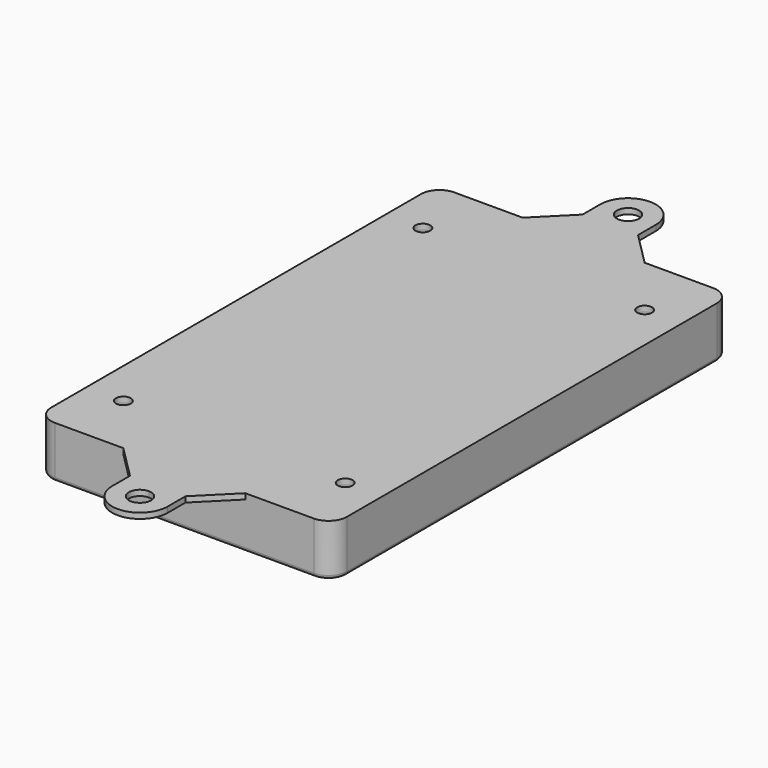
from build123d import *

# Parameters (mm, degrees)
F0_R      = 4
F1_DEPTH  = 25
F2_DEPTH  = 3
F3_DEPTH  = 18
F6_DEPTH  = 2
F8_DEPTH  = 20
F9_DEPTH  = 16
F10_DEPTH = 25
F7_R      = 6
F7_R_2    = 4
F11_DEPTH = 6
F13_DEPTH = 9
F14_R     = 3
F15_R     = 2
F16_R     = 4
F16_R_2   = 6
F17_DEPTH = 3


with BuildPart() as f1:
    # F0 (on Top) → F1 (new body)
    with BuildSketch(Plane.XY):
        with BuildLine():
            ThreePointArc((14.05, 38.3825811321), (16.9789321881, 31.3115133202), (24.05, 28.3825811321))
            Line((24.05, 28.3825811321), (164.05, 28.3825811321))
            ThreePointArc((164.05, 28.3825811321), (171.1210678119, 31.3115133202), (174.05, 38.3825811321))
            Line((174.05, 38.3825811321), (174.05, 288.3825811321))
            ThreePointArc((174.05, 288.3825811321), (171.1210678119, 295.4536489439), (164.05, 298.3825811321))
            Line((164.05, 298.3825811321), (24.05, 298.3825811321))
            ThreePointArc((24.05, 298.3825811321), (16.9789321881, 295.4536489439), (14.05, 288.3825811321))
            Line((14.05, 288.3825811321), (14.05, 38.3825811321))
        make_face()
        with Locations((34.05, 62.1325811321)):
            Circle(F0_R, mode=Mode.SUBTRACT)
        with Locations((154.05, 62.1325811321)):
            Circle(F0_R, mode=Mode.SUBTRACT)
        with Locations((34.05, 264.6325811321)):
            Circle(F0_R, mode=Mode.SUBTRACT)
        with BuildLine():
            ThreePointArc((30.05, 208.0453240566), (30.058730902, 208.5396812427), (30.0849127182, 209.033421831))
            ThreePointArc((30.0849127182, 209.033421831), (94.05, 268.6325811321), (158.0150872818, 209.033421831))
            ThreePointArc((158.0150872818, 209.033421831), (158.041269098, 208.5396812427), (158.05, 208.0453240566))
            Line((158.05, 208.0453240566), (158.05, 118.7198382075))
            ThreePointArc((158.05, 118.7198382075), (158.041269098, 118.2254810215), (158.0150872818, 117.7317404331))
            ThreePointArc((158.0150872818, 117.7317404331), (94.05, 58.1325811321), (30.0849127182, 117.7317404331))
            ThreePointArc((30.0849127182, 117.7317404331), (30.058730902, 118.2254810215), (30.05, 118.7198382075))
            Line((30.05, 118.7198382075), (30.05, 208.0453240566))
        make_face(mode=Mode.SUBTRACT)
        with Locations((154.05, 264.6325811321)):
            Circle(F0_R, mode=Mode.SUBTRACT)
        with BuildLine():
            ThreePointArc((158.0150872818, 209.033421831), (94.05, 268.6325811321), (30.0849127182, 209.033421831))
            ThreePointArc((30.0849127182, 209.033421831), (30.058730902, 208.5396812427), (30.05, 208.0453240566))
            Line((30.05, 208.0453240566), (30.05, 118.7198382075))
            ThreePointArc((30.05, 118.7198382075), (30.058730902, 118.2254810215), (30.0849127182, 117.7317404331))
            ThreePointArc((30.0849127182, 117.7317404331), (94.05, 58.1325811321), (158.0150872818, 117.7317404331))
            ThreePointArc((158.0150872818, 117.7317404331), (158.041269098, 118.2254810215), (158.05, 118.7198382075))
            Line((158.05, 118.7198382075), (158.05, 208.0453240566))
            ThreePointArc((158.05, 208.0453240566), (158.041269098, 208.5396812427), (158.0150872818, 209.033421831))
        make_face()
        with BuildLine():
            Line((34.05, 118.7198382075), (34.05, 208.0453240566))
            ThreePointArc((34.05, 208.0453240566), (34.0562363586, 208.3984363324), (34.0749376559, 208.7511081812))
            ThreePointArc((34.0749376559, 208.7511081812), (94.05, 264.6325811321), (154.0250623441, 208.7511081812))
            ThreePointArc((154.0250623441, 208.7511081812), (154.0437636414, 208.3984363324), (154.05, 208.0453240566))
            Line((154.05, 208.0453240566), (154.05, 118.7198382075))
            ThreePointArc((154.05, 118.7198382075), (154.0437636414, 118.3667259318), (154.0250623441, 118.0140540829))
            ThreePointArc((154.0250623441, 118.0140540829), (94.05, 62.1325811321), (34.0749376559, 118.0140540829))
            ThreePointArc((34.0749376559, 118.0140540829), (34.0562363586, 118.3667259318), (34.05, 118.7198382075))
        make_face(mode=Mode.SUBTRACT)
        with BuildLine():
            ThreePointArc((34.0749376559, 208.7511081812), (34.0562363586, 208.3984363324), (34.05, 208.0453240566))
            Line((34.05, 208.0453240566), (34.05, 118.7198382075))
            ThreePointArc((34.05, 118.7198382075), (34.0562363586, 118.3667259318), (34.0749376559, 118.0140540829))
            ThreePointArc((34.0749376559, 118.0140540829), (94.05, 62.1325811321), (154.0250623441, 118.0140540829))
            ThreePointArc((154.0250623441, 118.0140540829), (154.0437636414, 118.3667259318), (154.05, 118.7198382075))
            Line((154.05, 118.7198382075), (154.05, 208.0453240566))
            ThreePointArc((154.05, 208.0453240566), (154.0437636414, 208.3984363324), (154.0250623441, 208.7511081812))
            ThreePointArc((154.0250623441, 208.7511081812), (94.05, 264.6325811321), (34.0749376559, 208.7511081812))
        make_face()
        with BuildLine():
            ThreePointArc((151.0325436409, 208.5393729438), (151.045634549, 208.2925026496), (151.05, 208.0453240566))
            Line((151.05, 208.0453240566), (151.05, 118.7198382075))
            ThreePointArc((151.05, 118.7198382075), (151.045634549, 118.4726596145), (151.0325436409, 118.2257893203))
            ThreePointArc((151.0325436409, 118.2257893203), (94.05, 65.1325811321), (37.0674563591, 118.2257893203))
            ThreePointArc((37.0674563591, 118.2257893203), (37.054365451, 118.4726596145), (37.05, 118.7198382075))
            Line((37.05, 118.7198382075), (37.05, 208.0453240566))
            ThreePointArc((37.05, 208.0453240566), (37.054365451, 208.2925026496), (37.0674563591, 208.5393729438))
            ThreePointArc((37.0674563591, 208.5393729438), (94.05, 261.6325811321), (151.0325436409, 208.5393729438))
        make_face(mode=Mode.SUBTRACT)
        with BuildLine():
            Line((151.05, 118.7198382075), (151.05, 208.0453240566))
            ThreePointArc((151.05, 208.0453240566), (151.045634549, 208.2925026496), (151.0325436409, 208.5393729438))
            ThreePointArc((151.0325436409, 208.5393729438), (94.05, 261.6325811321), (37.0674563591, 208.5393729438))
            ThreePointArc((37.0674563591, 208.5393729438), (37.054365451, 208.2925026496), (37.05, 208.0453240566))
            Line((37.05, 208.0453240566), (37.05, 118.7198382075))
            ThreePointArc((37.05, 118.7198382075), (37.054365451, 118.4726596145), (37.0674563591, 118.2257893203))
            ThreePointArc((37.0674563591, 118.2257893203), (94.05, 65.1325811321), (151.0325436409, 118.2257893203))
            ThreePointArc((151.0325436409, 118.2257893203), (151.045634549, 118.4726596145), (151.05, 118.7198382075))
        make_face()
    extrude(amount=-F1_DEPTH)

    # F0 (on Top) → F2 (join)
    with BuildSketch(Plane.XY):
        with BuildLine():
            ThreePointArc((34.0749376559, 208.7511081812), (34.0562363586, 208.3984363324), (34.05, 208.0453240566))
            Line((34.05, 208.0453240566), (34.05, 118.7198382075))
            ThreePointArc((34.05, 118.7198382075), (34.0562363586, 118.3667259318), (34.0749376559, 118.0140540829))
            ThreePointArc((34.0749376559, 118.0140540829), (94.05, 62.1325811321), (154.0250623441, 118.0140540829))
            ThreePointArc((154.0250623441, 118.0140540829), (154.0437636414, 118.3667259318), (154.05, 118.7198382075))
            Line((154.05, 118.7198382075), (154.05, 208.0453240566))
            ThreePointArc((154.05, 208.0453240566), (154.0437636414, 208.3984363324), (154.0250623441, 208.7511081812))
            ThreePointArc((154.0250623441, 208.7511081812), (94.05, 264.6325811321), (34.0749376559, 208.7511081812))
        make_face()
        with BuildLine():
            ThreePointArc((151.0325436409, 208.5393729438), (151.045634549, 208.2925026496), (151.05, 208.0453240566))
            Line((151.05, 208.0453240566), (151.05, 118.7198382075))
            ThreePointArc((151.05, 118.7198382075), (151.045634549, 118.4726596145), (151.0325436409, 118.2257893203))
            ThreePointArc((151.0325436409, 118.2257893203), (94.05, 65.1325811321), (37.0674563591, 118.2257893203))
            ThreePointArc((37.0674563591, 118.2257893203), (37.054365451, 118.4726596145), (37.05, 118.7198382075))
            Line((37.05, 118.7198382075), (37.05, 208.0453240566))
            ThreePointArc((37.05, 208.0453240566), (37.054365451, 208.2925026496), (37.0674563591, 208.5393729438))
            ThreePointArc((37.0674563591, 208.5393729438), (94.05, 261.6325811321), (151.0325436409, 208.5393729438))
        make_face(mode=Mode.SUBTRACT)
    extrude(amount=F2_DEPTH)

    # F0 (on Top) → F3 (cut)
    with BuildSketch(Plane.XY):
        with BuildLine():
            Line((151.05, 118.7198382075), (151.05, 208.0453240566))
            ThreePointArc((151.05, 208.0453240566), (151.045634549, 208.2925026496), (151.0325436409, 208.5393729438))
            ThreePointArc((151.0325436409, 208.5393729438), (94.05, 261.6325811321), (37.0674563591, 208.5393729438))
            ThreePointArc((37.0674563591, 208.5393729438), (37.054365451, 208.2925026496), (37.05, 208.0453240566))
            Line((37.05, 208.0453240566), (37.05, 118.7198382075))
            ThreePointArc((37.05, 118.7198382075), (37.054365451, 118.4726596145), (37.0674563591, 118.2257893203))
            ThreePointArc((37.0674563591, 118.2257893203), (94.05, 65.1325811321), (151.0325436409, 118.2257893203))
            ThreePointArc((151.0325436409, 118.2257893203), (151.045634549, 118.4726596145), (151.05, 118.7198382075))
        make_face()
    extrude(amount=-F3_DEPTH, mode=Mode.SUBTRACT)

    # F4 (on face) → F5 (join, up to the next surface of F1)
    with BuildSketch(Plane.XY.offset(3)):
        with BuildLine():
            ThreePointArc((63.3, 70.0663530628), (65.1877495215, 64.9049197262), (69.9600985222, 62.1793597175))
            ThreePointArc((69.9600985222, 62.1793597175), (88.3, 60.6325811321), (106.6399014778, 62.1793597175))
            ThreePointArc((106.6399014778, 62.1793597175), (109.0997725506, 63.0263439319), (111.1577970177, 64.617847387))
            ThreePointArc((111.1577970177, 64.617847387), (98.7563887447, 62.3170645345), (86.1478631202, 62.6541260499))
            ThreePointArc((86.1478631202, 62.6541260499), (78.1937130529, 63.1086914432), (70.2950738916, 64.1511080538))
            ThreePointArc((70.2950738916, 64.1511080538), (66.9266219225, 65.9586086463), (65.3334610334, 69.4335712996))
            ThreePointArc((65.3334610334, 69.4335712996), (64.3111007877, 70.0023086838), (63.3, 70.5908304601))
            Line((63.3, 70.5908304601), (63.3, 70.0663530628))
        make_face()
        with BuildLine():
            ThreePointArc((107.5304157815, 66.7459245602), (109.1654742984, 67.168670617), (110.7873217221, 67.6395649966))
            ThreePointArc((110.7873217221, 67.6395649966), (111.1704314293, 68.826177739), (111.3, 70.0663530628))
            Line((111.3, 70.0663530628), (111.3, 135.1988092013))
            ThreePointArc((111.3, 135.1988092013), (109.8841878588, 139.0698842038), (106.3049261084, 141.1140542103))
            ThreePointArc((106.3049261084, 141.1140542103), (88.3, 142.6325811321), (70.2950738916, 141.1140542103))
            ThreePointArc((70.2950738916, 141.1140542103), (66.7158121412, 139.0698842038), (65.3, 135.1988092013))
            Line((65.3, 135.1988092013), (65.3, 72.8946079133))
            ThreePointArc((65.3, 72.8946079133), (66.2944325049, 72.3286907176), (67.3, 71.7828040152))
            Line((67.3, 71.7828040152), (67.3, 135.1988092013))
            ThreePointArc((67.3, 135.1988092013), (68.2438747608, 137.7795258696), (70.6300492611, 139.142305874))
            ThreePointArc((70.6300492611, 139.142305874), (88.3, 140.6325811321), (105.9699507389, 139.142305874))
            ThreePointArc((105.9699507389, 139.142305874), (108.3561252392, 137.7795258696), (109.3, 135.1988092013))
            Line((109.3, 135.1988092013), (109.3, 70.0663530628))
            ThreePointArc((109.3, 70.0663530628), (108.8299903064, 68.185085289), (107.5304157815, 66.7459245602))
        make_face()
        with BuildLine():
            ThreePointArc((67.3, 71.7828040152), (86.9533102792, 65.5751092381), (107.5304157815, 66.7459245602))
            ThreePointArc((107.5304157815, 66.7459245602), (108.8299903064, 68.185085289), (109.3, 70.0663530628))
            Line((109.3, 70.0663530628), (109.3, 135.1988092013))
            ThreePointArc((109.3, 135.1988092013), (108.3561252392, 137.7795258696), (105.9699507389, 139.142305874))
            ThreePointArc((105.9699507389, 139.142305874), (88.3, 140.6325811321), (70.6300492611, 139.142305874))
            ThreePointArc((70.6300492611, 139.142305874), (68.2438747608, 137.7795258696), (67.3, 135.1988092013))
            Line((67.3, 135.1988092013), (67.3, 71.7828040152))
        make_face()
        with BuildLine():
            Line((80.3, 100.1325811321), (102.3, 100.1325811321))
            ThreePointArc((102.3, 100.1325811321), (104.4213203436, 99.2539014756), (105.3, 97.1325811321))
            Line((105.3, 97.1325811321), (105.3, 95.1325811321))
            ThreePointArc((105.3, 95.1325811321), (104.4213203436, 93.0112607885), (102.3, 92.1325811321))
            ThreePointArc((102.3, 92.1325811321), (100.1786796564, 91.2539014756), (99.3, 89.1325811321))
            Line((99.3, 89.1325811321), (99.3, 75.1325811321))
            ThreePointArc((99.3, 75.1325811321), (98.4213203436, 73.0112607885), (96.3, 72.1325811321))
            Line((96.3, 72.1325811321), (80.3, 72.1325811321))
            ThreePointArc((80.3, 72.1325811321), (78.1786796564, 73.0112607885), (77.3, 75.1325811321))
            Line((77.3, 75.1325811321), (77.3, 97.1325811321))
            ThreePointArc((77.3, 97.1325811321), (78.1786796564, 99.2539014756), (80.3, 100.1325811321))
        make_face(mode=Mode.SUBTRACT)
        with BuildLine():
            ThreePointArc((80.3, 105.1325811321), (78.1786796564, 106.0112607885), (77.3, 108.1325811321))
            Line((77.3, 108.1325811321), (77.3, 130.1325811321))
            ThreePointArc((77.3, 130.1325811321), (78.1786796564, 132.2539014756), (80.3, 133.1325811321))
            Line((80.3, 133.1325811321), (96.3, 133.1325811321))
            ThreePointArc((96.3, 133.1325811321), (98.4213203436, 132.2539014756), (99.3, 130.1325811321))
            Line((99.3, 130.1325811321), (99.3, 116.1325811321))
            ThreePointArc((99.3, 116.1325811321), (100.1786796564, 114.0112607885), (102.3, 113.1325811321))
            ThreePointArc((102.3, 113.1325811321), (104.4213203436, 112.2539014756), (105.3, 110.1325811321))
            Line((105.3, 110.1325811321), (105.3, 108.1325811321))
            ThreePointArc((105.3, 108.1325811321), (104.4213203436, 106.0112607885), (102.3, 105.1325811321))
            Line((102.3, 105.1325811321), (80.3, 105.1325811321))
        make_face(mode=Mode.SUBTRACT)
    extrude(until=Until.NEXT, dir=(0, 0, -1))

    # F4 (on face) → F6 (cut)
    with BuildSketch(Plane.XY.offset(3)):
        with BuildLine():
            ThreePointArc((107.5304157815, 66.7459245602), (109.1654742984, 67.168670617), (110.7873217221, 67.6395649966))
            ThreePointArc((110.7873217221, 67.6395649966), (111.1704314293, 68.826177739), (111.3, 70.0663530628))
            Line((111.3, 70.0663530628), (111.3, 135.1988092013))
            ThreePointArc((111.3, 135.1988092013), (109.8841878588, 139.0698842038), (106.3049261084, 141.1140542103))
            ThreePointArc((106.3049261084, 141.1140542103), (88.3, 142.6325811321), (70.2950738916, 141.1140542103))
            ThreePointArc((70.2950738916, 141.1140542103), (66.7158121412, 139.0698842038), (65.3, 135.1988092013))
            Line((65.3, 135.1988092013), (65.3, 72.8946079133))
            ThreePointArc((65.3, 72.8946079133), (66.2944325049, 72.3286907176), (67.3, 71.7828040152))
            Line((67.3, 71.7828040152), (67.3, 135.1988092013))
            ThreePointArc((67.3, 135.1988092013), (68.2438747608, 137.7795258696), (70.6300492611, 139.142305874))
            ThreePointArc((70.6300492611, 139.142305874), (88.3, 140.6325811321), (105.9699507389, 139.142305874))
            ThreePointArc((105.9699507389, 139.142305874), (108.3561252392, 137.7795258696), (109.3, 135.1988092013))
            Line((109.3, 135.1988092013), (109.3, 70.0663530628))
            ThreePointArc((109.3, 70.0663530628), (108.8299903064, 68.185085289), (107.5304157815, 66.7459245602))
        make_face()
    extrude(amount=-F6_DEPTH, mode=Mode.SUBTRACT)

    # F7 (on face) → F8 (join)
    with BuildSketch(Plane(origin=(0, 0, -25), x_dir=(1, 0, 0), z_dir=(0, 0, -1))):
        with BuildLine():
            ThreePointArc((97.33842436, -163.3825811321), (110.8067035675, -149.9143019245), (124.274982775, -163.3825811321))
            Line((124.274982775, -163.3825811321), (129.274982775, -163.3825811321))
            ThreePointArc((129.274982775, -163.3825811321), (110.8067035675, -144.9143019245), (92.33842436, -163.3825811321))
            Line((92.33842436, -163.3825811321), (97.33842436, -163.3825811321))
        make_face()
        with BuildLine():
            Line((97.33842436, -163.3825811321), (124.274982775, -163.3825811321))
            ThreePointArc((124.274982775, -163.3825811321), (110.8067035675, -149.9143019245), (97.33842436, -163.3825811321))
        make_face()
        with BuildLine():
            ThreePointArc((97.33842436, -163.3825811321), (110.8067035675, -176.8508603396), (124.274982775, -163.3825811321))
            Line((124.274982775, -163.3825811321), (97.33842436, -163.3825811321))
        make_face()
        with BuildLine():
            Line((129.274982775, -163.3825811321), (124.274982775, -163.3825811321))
            ThreePointArc((124.274982775, -163.3825811321), (110.8067035675, -176.8508603396), (97.33842436, -163.3825811321))
            Line((97.33842436, -163.3825811321), (92.33842436, -163.3825811321))
            ThreePointArc((92.33842436, -163.3825811321), (110.8067035675, -181.8508603396), (129.274982775, -163.3825811321))
        make_face()
    extrude(amount=-F8_DEPTH)

    # F7 (on face) → F9 (cut)
    with BuildSketch(Plane(origin=(0, 0, -25), x_dir=(1, 0, 0), z_dir=(0, 0, -1))):
        with BuildLine():
            Line((97.33842436, -163.3825811321), (124.274982775, -163.3825811321))
            ThreePointArc((124.274982775, -163.3825811321), (110.8067035675, -149.9143019245), (97.33842436, -163.3825811321))
        make_face()
        with BuildLine():
            ThreePointArc((97.33842436, -163.3825811321), (110.8067035675, -176.8508603396), (124.274982775, -163.3825811321))
            Line((124.274982775, -163.3825811321), (97.33842436, -163.3825811321))
        make_face()
    extrude(amount=-F9_DEPTH, mode=Mode.SUBTRACT)

    # F7 (on face) → F10 (cut)
    with BuildSketch(Plane(origin=(0, 0, -25), x_dir=(1, 0, 0), z_dir=(0, 0, -1))):
        with BuildLine():
            Line((35.0181770675, -163.3825811321), (61.9547354825, -163.3825811321))
            ThreePointArc((61.9547354825, -163.3825811321), (48.486456275, -149.9143019245), (35.0181770675, -163.3825811321))
        make_face()
        with BuildLine():
            ThreePointArc((35.0181770675, -163.3825811321), (48.486456275, -176.8508603396), (61.9547354825, -163.3825811321))
            Line((61.9547354825, -163.3825811321), (35.0181770675, -163.3825811321))
        make_face()
    extrude(amount=-F10_DEPTH, mode=Mode.SUBTRACT)

    # F7 (on face) → F11 (cut)
    with BuildSketch(Plane(origin=(0, 0, -25), x_dir=(1, 0, 0), z_dir=(0, 0, -1))):
        with Locations((154.05, -264.6325811321)):
            Circle(F7_R)
        with Locations((154.05, -264.6325811321)):
            Circle(F7_R_2, mode=Mode.SUBTRACT)
        with Locations((34.05, -264.6325811321)):
            Circle(F7_R)
        with Locations((34.05, -264.6325811321)):
            Circle(F7_R_2, mode=Mode.SUBTRACT)
        with Locations((34.05, -62.1325811321)):
            Circle(F7_R)
        with Locations((34.05, -62.1325811321)):
            Circle(F7_R_2, mode=Mode.SUBTRACT)
        with Locations((154.05, -62.1325811321)):
            Circle(F7_R)
        with Locations((154.05, -62.1325811321)):
            Circle(F7_R_2, mode=Mode.SUBTRACT)
    extrude(amount=-F11_DEPTH, mode=Mode.SUBTRACT)

    # F12 (on face) → F13 (cut, through all)
    with BuildSketch(Plane(origin=(0, 0, -9), x_dir=(1, 0, 0), z_dir=(0, 0, -1))):
        with BuildLine():
            Line((99.3, -89.1325811321), (99.3, -100.1325811321))
            Line((99.3, -100.1325811321), (102.3, -100.1325811321))
            ThreePointArc((102.3, -100.1325811321), (104.4213203436, -99.2539014756), (105.3, -97.1325811321))
            Line((105.3, -97.1325811321), (105.3, -95.1325811321))
            ThreePointArc((105.3, -95.1325811321), (104.4213203436, -93.0112607885), (102.3, -92.1325811321))
            ThreePointArc((102.3, -92.1325811321), (100.1786796564, -91.2539014756), (99.3, -89.1325811321))
        make_face()
        with BuildLine():
            Line((102.3, -105.1325811321), (99.3, -105.1325811321))
            Line((99.3, -105.1325811321), (99.3, -116.1325811321))
            ThreePointArc((99.3, -116.1325811321), (100.1786796564, -114.0112607885), (102.3, -113.1325811321))
            ThreePointArc((102.3, -113.1325811321), (104.4213203436, -112.2539014756), (105.3, -110.1325811321))
            Line((105.3, -110.1325811321), (105.3, -108.1325811321))
            ThreePointArc((105.3, -108.1325811321), (104.4213203436, -106.0112607885), (102.3, -105.1325811321))
        make_face()
    extrude(amount=F13_DEPTH, mode=Mode.SUBTRACT)

    # F14
    f14_edges = [f1.edges().sort_by_distance(p)[0] for p in [
        (37.05, 137.494455, -18),
        (37.05, 189.270707, -18),
        (129.274983, 163.382581, -18),
        (45.560349, 92.057923, -18),
        (37.054365, 118.47266, -18),
        (37.054365, 208.292503, -18),
        (94.05, 261.632581, -18),
        (151.045635, 208.292503, -18),
        (151.05, 163.382581, -18),
        (151.045635, 118.47266, -18),
        (138.753424, 86.692578, -18),
    ]]
    fillet(f14_edges, radius=F14_R)

    # F15
    f15_edges = [f1.edges().sort_by_distance(p)[0] for p in [
        (94.05, 28.382581, -25),
        (14.05, 163.382581, -25),
        (16.978932, 295.453649, -25),
        (16.978932, 31.311513, -25),
        (94.05, 298.382581, -25),
        (171.121068, 295.453649, -25),
        (171.121068, 31.311513, -25),
        (174.05, 163.382581, -25),
    ]]
    fillet(f15_edges, radius=F15_R)

    # F16 (on face) → F17 (join, through all)
    with BuildSketch(Plane.XY):
        with BuildLine():
            Line((61.05, 298.3825811321), (24.05, 298.3825811321))
            ThreePointArc((24.05, 298.3825811321), (16.9789321881, 295.4536489439), (14.05, 288.3825811321))
            Line((14.05, 288.3825811321), (14.05, 38.3825811321))
            ThreePointArc((14.05, 38.3825811321), (16.9789321881, 31.3115133202), (24.05, 28.3825811321))
            Line((24.05, 28.3825811321), (61.05, 28.3825811321))
            Line((61.05, 28.3825811321), (94.05, 28.3825811321))
            Line((94.05, 28.3825811321), (127.05, 28.3825811321))
            Line((127.05, 28.3825811321), (164.05, 28.3825811321))
            ThreePointArc((164.05, 28.3825811321), (171.1210678119, 31.3115133202), (174.05, 38.3825811321))
            Line((174.05, 38.3825811321), (174.05, 288.3825811321))
            ThreePointArc((174.05, 288.3825811321), (171.1210678119, 295.4536489439), (164.05, 298.3825811321))
            Line((164.05, 298.3825811321), (127.05, 298.3825811321))
            Line((127.05, 298.3825811321), (61.05, 298.3825811321))
        make_face()
        with Locations((34.05, 62.1325811321)):
            Circle(F16_R, mode=Mode.SUBTRACT)
        with Locations((154.05, 62.1325811321)):
            Circle(F16_R, mode=Mode.SUBTRACT)
        with Locations((34.05, 264.6325811321)):
            Circle(F16_R, mode=Mode.SUBTRACT)
        with Locations((154.05, 264.6325811321)):
            Circle(F16_R, mode=Mode.SUBTRACT)
        with BuildLine():
            Line((79.05, 316.3825811321), (61.05, 298.3825811321))
            Line((61.05, 298.3825811321), (127.05, 298.3825811321))
            Line((127.05, 298.3825811321), (109.05, 316.3825811321))
            Line((109.05, 316.3825811321), (109.05, 328.3825811321))
            ThreePointArc((109.05, 328.3825811321), (94.05, 343.3825811321), (79.05, 328.3825811321))
            Line((79.05, 328.3825811321), (79.05, 316.3825811321))
        make_face()
        with Locations((94.05, 328.3825811321)):
            Circle(F16_R_2, mode=Mode.SUBTRACT)
        with BuildLine():
            Line((94.05, 28.3825811321), (61.05, 28.3825811321))
            Line((61.05, 28.3825811321), (79.05, 10.3825811321))
            Line((79.05, 10.3825811321), (79.05, -1.6174188679))
            ThreePointArc((79.05, -1.6174188679), (94.05, -16.6174188679), (109.05, -1.6174188679))
            Line((109.05, -1.6174188679), (109.05, 10.3825811321))
            Line((109.05, 10.3825811321), (127.05, 28.3825811321))
            Line((127.05, 28.3825811321), (94.05, 28.3825811321))
        make_face()
        with BuildLine():
            ThreePointArc((100.05, -1.6174188679), (89.8073593129, -5.8600595551), (94.05, 4.3825811321))
            ThreePointArc((94.05, 4.3825811321), (98.2926406871, 2.6252218192), (100.05, -1.6174188679))
        make_face(mode=Mode.SUBTRACT)
    extrude(amount=F17_DEPTH)


solid = f1.part
